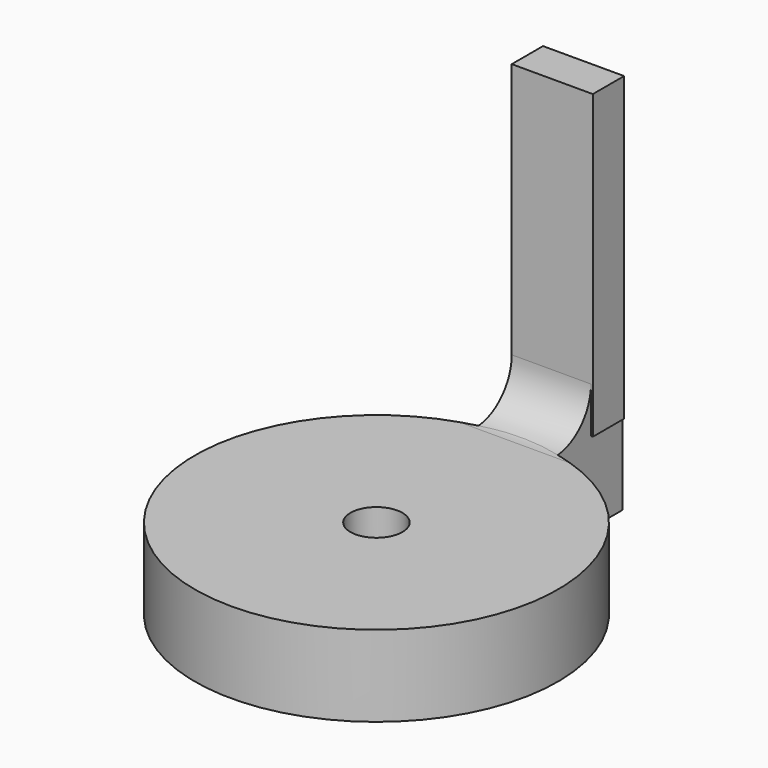
from build123d import *

# Parameters (mm, degrees)
F0_R        = 19.84
F1_DEPTH    = 8.86
F2_W        = 8.66
F2_H        = 8.8
F3_DEPTH    = 8.86
F4_W        = 8.86
F4_H        = 4.27
F5_DEPTH    = 32.96
F6_R        = 2.84
F7_DEPTH    = 8.86
F8_T1_DEPTH = 8.66
F8_T6_DEPTH = 33.66
F8_S7_R     = 19.84
F8_T8_DEPTH = 19


# Not quite as in the source:
# - a fillet or chamfer that OpenCascade refuses, or shapes differently, is made with other operations: its cross-section is extruded or revolved along the edge and cut away or added


with BuildPart() as f1:
    # F0 (on Top) → F1 (new body)
    with BuildSketch(Plane.XY):
        Circle(F0_R)
    extrude(amount=F1_DEPTH)

    # F2 (on Top) → F3 (join)
    with BuildSketch(Plane.XY):
        with Locations((0, 23.761732877)):
            Rectangle(F2_W, F2_H)
    extrude(amount=F3_DEPTH)

    # F4 (on face) → F5 (join)
    with BuildSketch(Plane.XY.offset(8.86)):
        with Locations((0.1, 26.026732877)):
            Rectangle(F4_W, F4_H)
    extrude(amount=F5_DEPTH)

    # F6 (on face) → F7 (cut, through all)
    with BuildSketch(Plane.XY.offset(8.86)):
        Circle(F6_R)
    extrude(amount=-F7_DEPTH, mode=Mode.SUBTRACT)

    # F8: fillet of radius 5 on 1 edges, made by hand

    # F8_s2 → F8_t1 (join)
    with BuildSketch(Plane.YZ.offset(-4.33)):
        with BuildLine():
            ThreePointArc((18.891732877, 8.86), (22.4272667829, 10.3244660941), (23.891732877, 13.86))
            Line((23.891732877, 13.86), (23.891732877, 8.86))
            Line((23.891732877, 8.86), (18.891732877, 8.86))
        make_face()
    extrude(amount=F8_T1_DEPTH)


with BuildPart() as f8_tool4:
    # F8_s5 → F8_t6 (new body)
    with BuildSketch(Plane.YZ.offset(-16.83)):
        with BuildLine():
            ThreePointArc((18.891732877, 8.86), (22.4272667829, 10.3244660941), (23.891732877, 13.86))
            Line((23.891732877, 13.86), (23.891732877, 8.86))
            Line((23.891732877, 8.86), (18.891732877, 8.86))
        make_face()
    extrude(amount=F8_T6_DEPTH)

    # F8_s7 → F8_t8 (intersect, symmetric)
    with BuildSketch(Plane.XY.offset(11.4)):
        Circle(F8_S7_R)
    extrude(amount=F8_T8_DEPTH, both=True, mode=Mode.INTERSECT)


with BuildPart() as f1_1:
    add(f1.part)

    # F8_t3: union F8_tool4
    add(f8_tool4.part)


solid = f1_1.part
